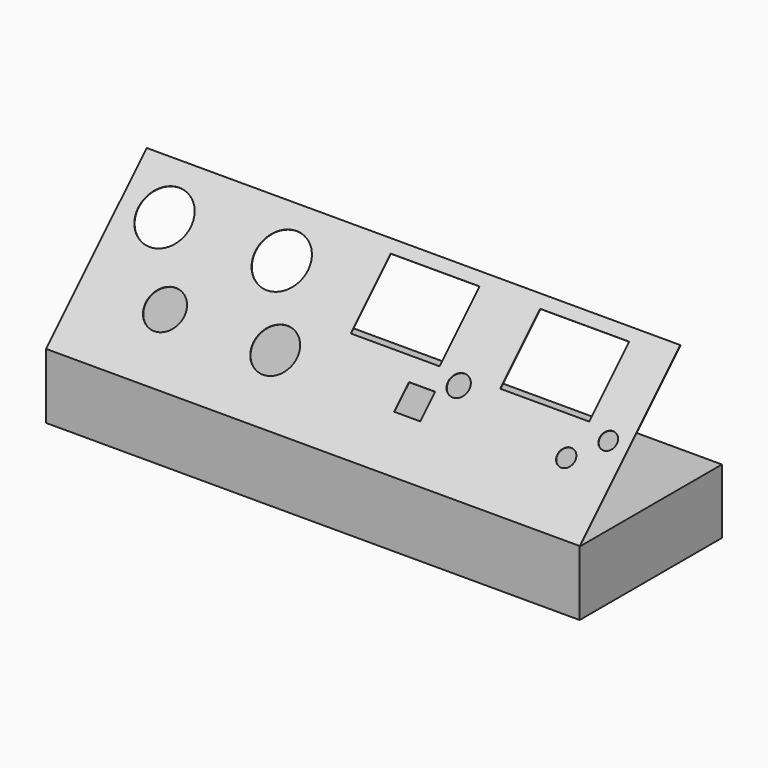
from build123d import *

# Parameters (mm, degrees)
F1_DEPTH = 209.55
F2_W     = 20.6375
F2_H     = 20.6375
F2_W_2   = 69.85
F2_H_2   = 55.5625
F3_DEPTH = 0.4064


# Not quite as in the source:
# - the dataset's text gives a spline's control points without its knots; the knots are read off the source's solid


with BuildPart() as f1:
    # F0 (on Right) → F1 (new body, symmetric)
    with BuildSketch(Plane.YZ):
        Polygon((-139.7, 0), (0, 0), (0, 50.8), (-139.2936, 50.8), (-139.2936, 51.054), (-40.6298144724, 149.7177855276), (-40.9171826682, 150.0051537235), (-139.7, 51.2223363917), align=None)
    extrude(amount=F1_DEPTH, both=True)

    # F2 (on face) → F3 (cut, through all)
    with BuildSketch(Plane(origin=(0, -95.4611681959, 95.4611681959), x_dir=(1, 0, 0), z_dir=(0, -0.7071067812, 0.7071067812))):
        with Locations((52.3081513166, -13.6913588034)):
            Rectangle(F2_W, F2_H)
        with Locations((139.6206513166, 40.2836411966)):
            Rectangle(F2_W_2, F2_H_2)
        with Locations((22.1456513166, 40.2836411966)):
            Rectangle(F2_W_2, F2_H_2)
        with BuildLine():
            add(Edge.make_bspline(
                [(-69.2965076834, -25.7584924034), (-66.1370016834, -28.9176682034), (-61.6969800834, -30.7569838034), (-57.2293486834, -30.7569838034), (-52.7614378834, -30.7569838034), (-48.3210606834, -28.9176682034), (-45.1618848834, -25.7584924034), (-42.0027344834, -22.5993420034), (-40.1637236834, -18.1593204034), (-40.1637236834, -13.6913588034), (-40.1637236834, -9.2234226034), (-42.0027344834, -4.7833502034), (-45.1618848834, -1.6242252034), (-48.3210606834, 1.5349251966), (-52.7614378834, 3.3742661966), (-57.2293486834, 3.3742661966)],
                knots=[3, 3, 3, 3, 4, 4, 4, 5, 5, 5, 6, 6, 6, 7, 7, 7, 8, 8, 8, 8], degree=3))
            add(Edge.make_bspline(
                [(-57.2293486834, 3.3742661966), (-61.6969800834, 3.3742661966), (-66.1370016834, 1.5349251966), (-69.2965076834, -1.6242252034)],
                knots=[0, 0, 0, 0, 1, 1, 1, 1], degree=3))
            add(Edge.make_bspline(
                [(-69.2965076834, -1.6242252034), (-72.4556326834, -4.7833502034), (-74.2949736834, -9.2234226034), (-74.2949736834, -13.6913588034), (-74.2949736834, -18.1593204034), (-72.4556326834, -22.5993420034), (-69.2965076834, -25.7584924034)],
                knots=[1, 1, 1, 1, 2, 2, 2, 3, 3, 3, 3], degree=3))
        make_face()
        with BuildLine():
            add(Edge.make_bspline(
                [(82.0141371166, 11.2521523966), (80.4710871166, 12.7948975966), (78.3027399166, 13.6930161966), (76.1206513166, 13.6930161966)],
                knots=[7, 7, 7, 7, 8, 8, 8, 8], degree=3))
            add(Edge.make_bspline(
                [(76.1206513166, 13.6930161966), (73.9388421166, 13.6930161966), (71.7701901166, 12.7948975966), (70.2274449166, 11.2521523966)],
                knots=[0, 0, 0, 0, 1, 1, 1, 1], degree=3))
            add(Edge.make_bspline(
                [(70.2274449166, 11.2521523966), (68.6847505166, 9.7091023966), (67.7862763166, 7.5404503966), (67.7862763166, 5.3586411966), (67.7862763166, 3.1768573966), (68.6847505166, 1.0081545966), (70.2274449166, -0.5345398034)],
                knots=[1, 1, 1, 1, 2, 2, 2, 3, 3, 3, 3], degree=3))
            add(Edge.make_bspline(
                [(70.2274449166, -0.5345398034), (71.7701901166, -2.0775898034), (73.9388421166, -2.9757338034), (76.1206513166, -2.9757338034), (78.3027399166, -2.9757338034), (80.4710871166, -2.0775898034), (82.0141371166, -0.5345398034)],
                knots=[3, 3, 3, 3, 4, 4, 4, 5, 5, 5, 5], degree=3))
            add(Edge.make_bspline(
                [(82.0141371166, -0.5345398034), (83.5572379166, 1.0081545966), (84.4550263166, 3.1768573966), (84.4550263166, 5.3586411966), (84.4550263166, 7.5404503966), (83.5572379166, 9.7091023966), (82.0141371166, 11.2521523966)],
                knots=[5, 5, 5, 5, 6, 6, 6, 7, 7, 7, 7], degree=3))
        make_face()
        with BuildLine():
            add(Edge.make_bspline(
                [(-68.0362866834, 54.8767285966), (-71.8565482834, 58.6969901966), (-77.2264130834, 60.9211411966), (-82.6293486834, 60.9211411966)],
                knots=[7, 7, 7, 7, 8, 8, 8, 8], degree=3))
            add(Edge.make_bspline(
                [(-82.6293486834, 60.9211411966), (-88.0319794834, 60.9211411966), (-93.4014886834, 58.6969901966), (-97.2220804834, 54.8767285966)],
                knots=[0, 0, 0, 0, 1, 1, 1, 1], degree=3))
            add(Edge.make_bspline(
                [(-97.2220804834, 54.8767285966), (-101.0426976834, 51.0561113966), (-103.2668486834, 45.6865767966), (-103.2668486834, 40.2836411966), (-103.2668486834, 34.8807055966), (-101.0426976834, 29.5111455966), (-97.2220804834, 25.6905791966)],
                knots=[1, 1, 1, 1, 2, 2, 2, 3, 3, 3, 3], degree=3))
            add(Edge.make_bspline(
                [(-97.2220804834, 25.6905791966), (-93.4014886834, 21.8703175966), (-88.0319794834, 19.6461411966), (-82.6293486834, 19.6461411966), (-77.2264130834, 19.6461411966), (-71.8565482834, 21.8703175966), (-68.0362866834, 25.6905791966)],
                knots=[3, 3, 3, 3, 4, 4, 4, 5, 5, 5, 5], degree=3))
            add(Edge.make_bspline(
                [(-68.0362866834, 25.6905791966), (-64.2160250834, 29.5111455966), (-61.9918486834, 34.8807055966), (-61.9918486834, 40.2836411966), (-61.9918486834, 45.6865767966), (-64.2160250834, 51.0561113966), (-68.0362866834, 54.8767285966)],
                knots=[5, 5, 5, 5, 6, 6, 6, 7, 7, 7, 7], degree=3))
        make_face()
        with BuildLine():
            add(Edge.make_bspline(
                [(-160.1112866834, 54.8767285966), (-163.9315482834, 58.6969901966), (-169.3014130834, 60.9211411966), (-174.7043486834, 60.9211411966)],
                knots=[7, 7, 7, 7, 8, 8, 8, 8], degree=3))
            add(Edge.make_bspline(
                [(-174.7043486834, 60.9211411966), (-180.1069794834, 60.9211411966), (-185.4764886834, 58.6969901966), (-189.2970804834, 54.8767285966)],
                knots=[0, 0, 0, 0, 1, 1, 1, 1], degree=3))
            add(Edge.make_bspline(
                [(-189.2970804834, 54.8767285966), (-193.1176976834, 51.0561113966), (-195.3418486834, 45.6865767966), (-195.3418486834, 40.2836411966), (-195.3418486834, 34.8807055966), (-193.1176976834, 29.5111455966), (-189.2970804834, 25.6905791966)],
                knots=[1, 1, 1, 1, 2, 2, 2, 3, 3, 3, 3], degree=3))
            add(Edge.make_bspline(
                [(-189.2970804834, 25.6905791966), (-185.4764886834, 21.8703175966), (-180.1069794834, 19.6461411966), (-174.7043486834, 19.6461411966), (-169.3014130834, 19.6461411966), (-163.9315482834, 21.8703175966), (-160.1112866834, 25.6905791966)],
                knots=[3, 3, 3, 3, 4, 4, 4, 5, 5, 5, 5], degree=3))
            add(Edge.make_bspline(
                [(-160.1112866834, 25.6905791966), (-156.2910250834, 29.5111455966), (-154.0668486834, 34.8807055966), (-154.0668486834, 40.2836411966), (-154.0668486834, 45.6865767966), (-156.2910250834, 51.0561113966), (-160.1112866834, 54.8767285966)],
                knots=[5, 5, 5, 5, 6, 6, 6, 7, 7, 7, 7], degree=3))
        make_face()
        with BuildLine():
            add(Edge.make_bspline(
                [(-133.1194686834, -3.0270418034), (-135.9113858834, -0.2354802034), (-139.8353556834, 1.3898911966), (-143.7837856834, 1.3898911966)],
                knots=[7, 7, 7, 7, 8, 8, 8, 8], degree=3))
            add(Edge.make_bspline(
                [(-143.7837856834, 1.3898911966), (-147.7318600834, 1.3898911966), (-151.6558044834, -0.2354802034), (-154.4477216834, -3.0270418034)],
                knots=[0, 0, 0, 0, 1, 1, 1, 1], degree=3))
            add(Edge.make_bspline(
                [(-154.4477216834, -3.0270418034), (-157.2396388834, -5.8189844034), (-158.8650356834, -9.7429288034), (-158.8650356834, -13.6913588034), (-158.8650356834, -17.6397888034), (-157.2396388834, -21.5637332034), (-154.4477216834, -24.3552948034)],
                knots=[1, 1, 1, 1, 2, 2, 2, 3, 3, 3, 3], degree=3))
            add(Edge.make_bspline(
                [(-154.4477216834, -24.3552948034), (-151.6558044834, -27.1472120034), (-147.7318600834, -28.7726088034), (-143.7837856834, -28.7726088034), (-139.8353556834, -28.7726088034), (-135.9113858834, -27.1472120034), (-133.1194686834, -24.3552948034), (-130.3279070834, -21.5637332034), (-128.7025356834, -17.6397888034), (-128.7025356834, -13.6913588034), (-128.7025356834, -9.7429288034), (-130.3279070834, -5.8189844034), (-133.1194686834, -3.0270418034)],
                knots=[3, 3, 3, 3, 4, 4, 4, 5, 5, 5, 6, 6, 6, 7, 7, 7, 7], degree=3))
        make_face()
        with BuildLine():
            add(Edge.make_bspline(
                [(176.2819699166, -8.7803704034), (174.9962473166, -7.4946732034), (173.1889611166, -6.7460336034), (171.3706513166, -6.7460336034)],
                knots=[7, 7, 7, 7, 8, 8, 8, 8], degree=3))
            add(Edge.make_bspline(
                [(171.3706513166, -6.7460336034), (169.5523161166, -6.7460336034), (167.7453601166, -7.4946732034), (166.4596629166, -8.7803704034)],
                knots=[0, 0, 0, 0, 1, 1, 1, 1], degree=3))
            add(Edge.make_bspline(
                [(166.4596629166, -8.7803704034), (165.1739657166, -10.0660930034), (164.4253261166, -11.8730236034), (164.4253261166, -13.6913588034), (164.4253261166, -15.5096686034), (165.1739657166, -17.3166246034), (166.4596629166, -18.6023218034)],
                knots=[1, 1, 1, 1, 2, 2, 2, 3, 3, 3, 3], degree=3))
            add(Edge.make_bspline(
                [(166.4596629166, -18.6023218034), (167.7453601166, -19.8880444034), (169.5523161166, -20.6366586034), (171.3706513166, -20.6366586034), (173.1889611166, -20.6366586034), (174.9962473166, -19.8880444034), (176.2819699166, -18.6023218034), (177.5676671166, -17.3166246034), (178.3159511166, -15.5096686034), (178.3159511166, -13.6913588034), (178.3159511166, -11.8730236034), (177.5676671166, -10.0660930034), (176.2819699166, -8.7803704034)],
                knots=[3, 3, 3, 3, 4, 4, 4, 5, 5, 5, 6, 6, 6, 7, 7, 7, 7], degree=3))
        make_face()
        with BuildLine():
            add(Edge.make_bspline(
                [(198.3663809166, 10.1293961966), (197.1175645166, 11.3782633966), (195.3622721166, 12.1055161966), (193.5956513166, 12.1055161966)],
                knots=[7, 7, 7, 7, 8, 8, 8, 8], degree=3))
            add(Edge.make_bspline(
                [(193.5956513166, 12.1055161966), (191.8293607166, 12.1055161966), (190.0740683166, 11.3782633966), (188.8248709166, 10.1293961966)],
                knots=[0, 0, 0, 0, 1, 1, 1, 1], degree=3))
            add(Edge.make_bspline(
                [(188.8248709166, 10.1293961966), (187.5760037166, 8.8805797966), (186.8487763166, 7.1249317966), (186.8487763166, 5.3586411966), (186.8487763166, 3.5923251966), (187.5760037166, 1.8367279966), (188.8248709166, 0.5878607966)],
                knots=[1, 1, 1, 1, 2, 2, 2, 3, 3, 3, 3], degree=3))
            add(Edge.make_bspline(
                [(188.8248709166, 0.5878607966), (190.0740683166, -0.6609810034), (191.8293607166, -1.3882338034), (193.5956513166, -1.3882338034), (195.3622721166, -1.3882338034), (197.1175645166, -0.6609810034), (198.3663809166, 0.5878607966)],
                knots=[3, 3, 3, 3, 4, 4, 4, 5, 5, 5, 5], degree=3))
            add(Edge.make_bspline(
                [(198.3663809166, 0.5878607966), (199.6155783166, 1.8367279966), (200.3425263166, 3.5923251966), (200.3425263166, 5.3586411966), (200.3425263166, 7.1249317966), (199.6155783166, 8.8805797966), (198.3663809166, 10.1293961966)],
                knots=[5, 5, 5, 5, 6, 6, 6, 7, 7, 7, 7], degree=3))
        make_face()
    extrude(amount=-F3_DEPTH, mode=Mode.SUBTRACT)


solid = f1.part
